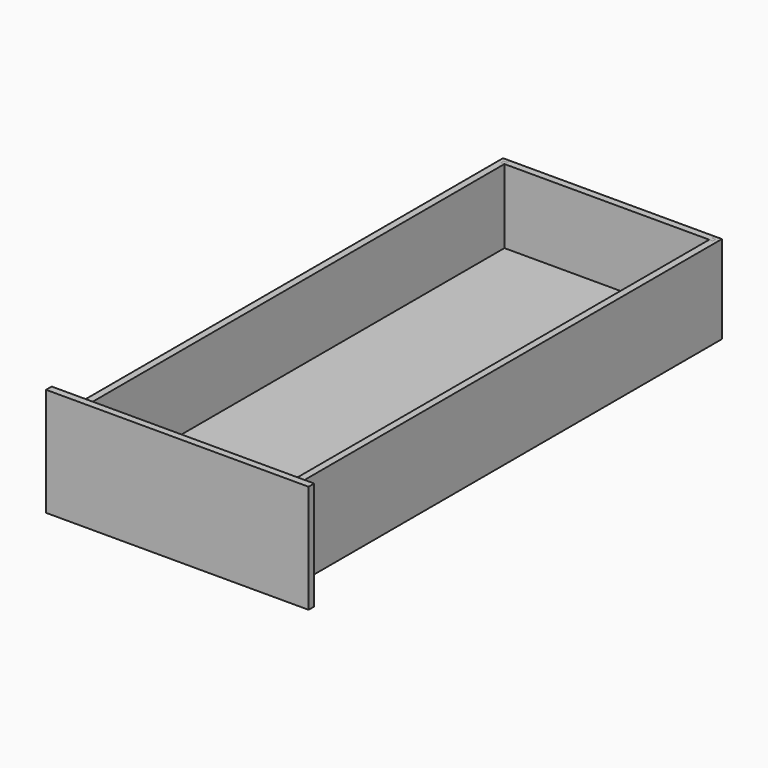
from build123d import *

# Parameters (mm, degrees)
F1_DEPTH  = 200
F2_DEPTH  = 200
F3_DEPTH  = 200
F4_DEPTH  = 200
F5_DEPTH  = 32
F7_DEPTH  = 561
F9_DEPTH  = 1211
F10_W     = 596
F10_H     = 246
F10_W_2   = 465.0000002384
F10_H_2   = 200
F10_W_3   = 16
F10_W_4   = 15.9999997616
F11_DEPTH = 16


with BuildPart() as f1:
    # F0 (on Top) → F1 (new body)
    with BuildSketch(Plane.XY):
        Polygon((-248.5, -609.5), (-232.5000002384, -609.5), (-232.5000002384, -601.5000002384), (-240.5000002384, -601.5000002384), (-240.5000002384, -593.5000002384), (-232.5000002384, -593.5000002384), (-232.5000002384, 593.5000002384), (-240.5000002384, 593.5000002384), (-240.5000002384, 601.5000002384), (-232.5000002384, 601.5000002384), (-232.5000002384, 609.5), (-248.5, 609.5), align=None)
    extrude(amount=F1_DEPTH)


with BuildPart() as f2:
    # F0 (on Top) → F2 (new body)
    with BuildSketch(Plane.XY):
        Polygon((232.5, -609.5), (248.5, -609.5), (248.5, 609.5), (232.5, 609.5), (232.5, 601.5000002384), (240.5, 601.5000002384), (240.5, 593.5000002384), (232.5, 593.5000002384), (232.5, -593.5000002384), (240.5, -593.5000002384), (240.5, -601.5000002384), (232.5, -601.5000002384), align=None)
    extrude(amount=F2_DEPTH)


with BuildPart() as f3:
    # F0 (on Top) → F3 (new body)
    with BuildSketch(Plane.XY):
        Polygon((232.5, 601.5000002384), (232.5, 609.5), (-232.5000002384, 609.5), (-232.5000002384, 601.5000002384), (-240.5000002384, 601.5000002384), (-240.5000002384, 593.5000002384), (-232.5000002384, 593.5000002384), (232.5, 593.5000002384), (240.5, 593.5000002384), (240.5, 601.5000002384), align=None)
    extrude(amount=F3_DEPTH)

    # F0 (on Top) → F5 (cut)
    with BuildSketch(Plane.XY):
        Polygon((232.5, 601.5000002384), (232.5, 609.5), (-232.5000002384, 609.5), (-232.5000002384, 601.5000002384), (-240.5000002384, 601.5000002384), (-240.5000002384, 593.5000002384), (-232.5000002384, 593.5000002384), (232.5, 593.5000002384), (240.5, 593.5000002384), (240.5, 601.5000002384), align=None)
    extrude(amount=F5_DEPTH, mode=Mode.SUBTRACT)


with BuildPart() as f4:
    # F0 (on Top) → F4 (new body)
    with BuildSketch(Plane.XY):
        Polygon((-232.5000002384, -609.5), (232.5, -609.5), (232.5, -601.5000002384), (240.5, -601.5000002384), (240.5, -593.5000002384), (232.5, -593.5000002384), (-232.5000002384, -593.5000002384), (-240.5000002384, -593.5000002384), (-240.5000002384, -601.5000002384), (-232.5000002384, -601.5000002384), align=None)
    extrude(amount=F4_DEPTH)


with BuildPart() as f7:
    # F6 (on face) → F7 (new body)
    with BuildSketch(Plane(origin=(0, 609.5, 0), x_dir=(-1, 0, 0), z_dir=(0, 1, 0))):
        Polygon((-232.5, 32), (-240.5, 32), (-240.5, 16), (240.5000002384, 16), (240.5000002384, 32), (232.5000002384, 32), align=None)
    extrude(amount=-F7_DEPTH)


with BuildPart() as f2_1:
    add(f2.part)

    # F8: cut F7
    add(f7.part, mode=Mode.SUBTRACT)


with BuildPart() as f1_1:
    add(f1.part)

    # F8: cut F7
    add(f7.part, mode=Mode.SUBTRACT)


with BuildPart() as f4_1:
    add(f4.part)

    # F8: cut F7
    add(f7.part, mode=Mode.SUBTRACT)


with BuildPart() as f9:
    # F6 (on face) → F9 (new body)
    with BuildSketch(Plane(origin=(0, 609.5, 0), x_dir=(-1, 0, 0), z_dir=(0, 1, 0))):
        Polygon((-232.5, 32), (-240.5, 32), (-240.5, 16), (240.5000002384, 16), (240.5000002384, 32), (232.5000002384, 32), align=None)
    extrude(amount=-F9_DEPTH)


with BuildPart() as f11:
    # F10 (on face) → F11 (new body)
    with BuildSketch(Plane.XZ.offset(609.5)):
        with Locations((0, 100)):
            Rectangle(F10_W, F10_H)
        Polygon((-248.5, 0), (-248.5, 200), (-232.5000002384, 200), (232.5, 200), (248.5, 200), (248.5, 0), (232.5, 0), (-232.5000002384, 0), align=None, mode=Mode.SUBTRACT)
        with Locations((-1.192e-07, 100)):
            Rectangle(F10_W_2, F10_H_2)
        with Locations((240.5, 100)):
            Rectangle(F10_W_3, F10_H_2)
        with Locations((-240.5000001192, 100)):
            Rectangle(F10_W_4, F10_H_2)
    extrude(amount=F11_DEPTH)


solid = Compound([f3.part, f2_1.part, f1_1.part, f4_1.part, f9.part, f11.part])
